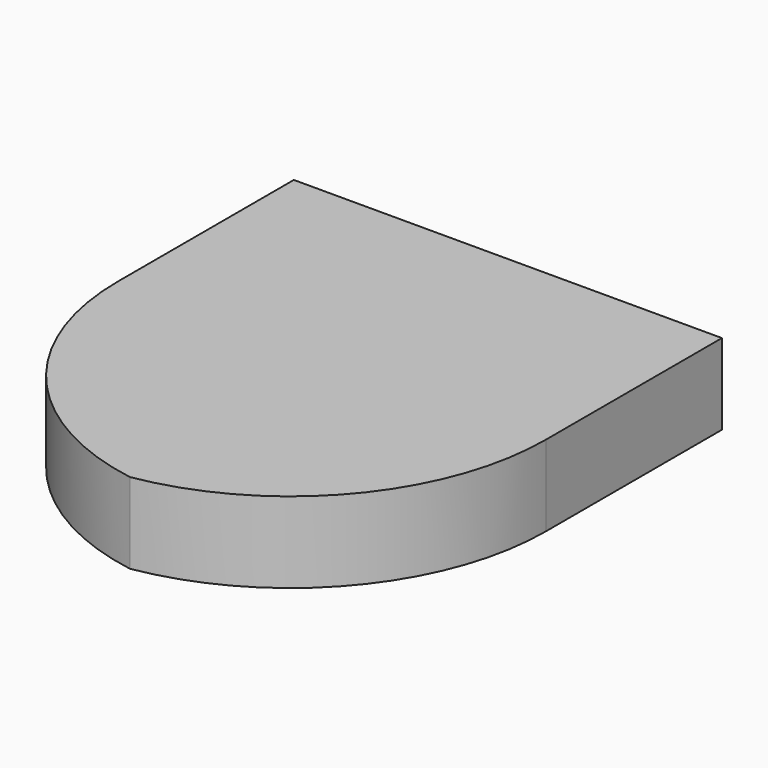
from build123d import *

# Parameters (mm, degrees)
F0_W        = 64.6526291966
F0_H        = 71.8573257327
F1_DEPTH    = 12.192
F2_T1_DEPTH = 205.3532271255


# Not quite as in the source:
# - a fillet or chamfer that OpenCascade refuses, or shapes differently, is made with other operations: its cross-section is extruded or revolved along the edge and cut away or added


with BuildPart() as f1:
    # F0 (on Top) → F1 (new body)
    with BuildSketch(Plane.XY):
        with Locations((7.299490273, 7.4890889227)):
            Rectangle(F0_W, F0_H)
    extrude(amount=F1_DEPTH)

    # F2: fillet of radius 38.6322454251 on 2 edges, made by hand

    # F2_s2 → F2_t1 (cut)
    with BuildSketch(Plane.XY.offset(-96.5806135627)):
        with BuildLine():
            ThreePointArc((0.9935594462, -28.4395739436), (28.3106821588, -17.1244512311), (39.6258048713, 10.1926714815))
            Line((39.6258048713, 10.1926714815), (39.6258048713, -28.4395739436))
            Line((39.6258048713, -28.4395739436), (0.9935594462, -28.4395739436))
        make_face()
        with BuildLine():
            ThreePointArc((-25.0268243253, 10.1926714815), (-13.7117016128, -17.1244512311), (13.6054210998, -28.4395739436))
            Line((13.6054210998, -28.4395739436), (-25.0268243253, -28.4395739436))
            Line((-25.0268243253, -28.4395739436), (-25.0268243253, 10.1926714815))
        make_face()
    extrude(amount=F2_T1_DEPTH, mode=Mode.SUBTRACT)


solid = f1.part
